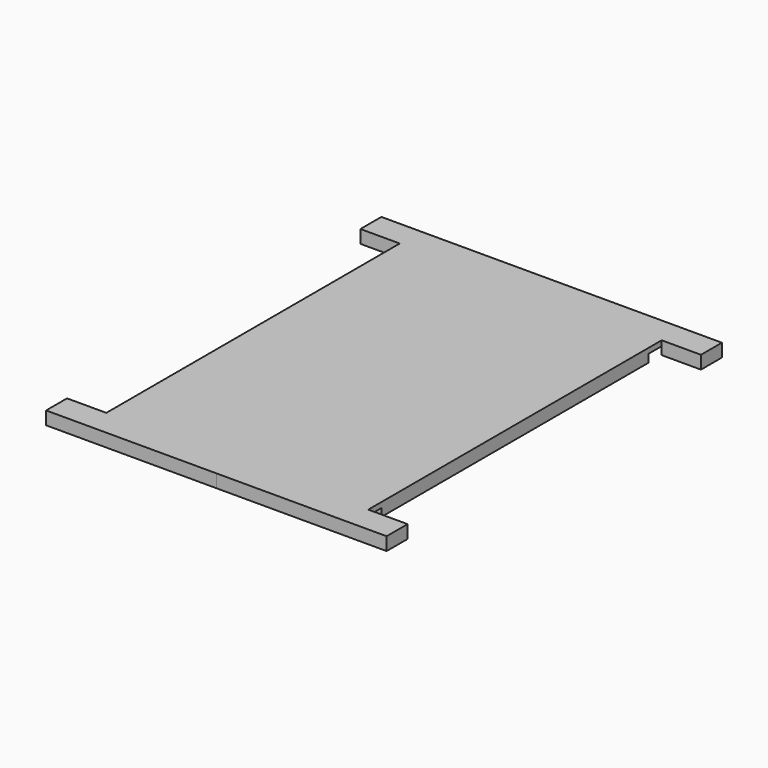
from build123d import *

# Parameters (mm, degrees)
F0_W     = 100
F0_H     = 127.2998210043
F1_DEPTH = 5
F2_DEPTH = 3
F3_DEPTH = 3


# Not quite as in the source:
# - ends of sketch curves that miss each other by under 0.0002 mm in the source are joined
# - a pattern or mirror of a feature is missing from the dataset's text; its kind, count and spacing are read off the source's solid


with BuildPart() as f1:
    # F0 (on Top) → F1 (new body)
    with BuildSketch(Plane.XY):
        Polygon((-65, 132.1264296972), (-65, 122.1264296972), (-50, 122.1264296972), (-50, 126.4795800469), (50, 126.4795800469), (50, 122.1264134925), (65, 122.1263972878), (65, 132.1264296972), (0, 132.1264266705), align=None)
        Polygon((-50, 126.4795800469), (-50, 122.1264296972), (-50, 115.7763972878), (50, 115.7763972878), (50, 122.1264296972), (50, 126.4795800469), align=None)
        with Locations((0, 52.1264867857)):
            Rectangle(F0_W, F0_H)
        Polygon((50, -11.5234237164), (-50, -11.5234237164), (-50, -17.8735703028), (-50, -21.843858043), (50, -21.843858043), (50, -17.8734237164), align=None)
    extrude(amount=F1_DEPTH)

    # F1_copies: F1 across plane


with BuildPart() as f1_1:
    add(f1.part)
    add(f1.part.mirror(Plane(origin=(-2e-06, 52.126426, 0), x_dir=(0, 0, -1), z_dir=(0, -1, 0))))

    # F0 (on Top) → F2 (cut)
    with BuildSketch(Plane.XY):
        Polygon((50, -11.5234237164), (-50, -11.5234237164), (-50, -17.8735703028), (-50, -21.843858043), (50, -21.843858043), (50, -17.8734237164), align=None)
    extrude(amount=F2_DEPTH, mode=Mode.SUBTRACT)

    # F0 (on Top) → F3 (cut)
    with BuildSketch(Plane.XY):
        Polygon((-50, 126.4795800469), (-50, 122.1264296972), (-50, 115.7763972878), (50, 115.7763972878), (50, 122.1264296972), (50, 126.4795800469), align=None)
    extrude(amount=F3_DEPTH, mode=Mode.SUBTRACT)


solid = f1_1.part
